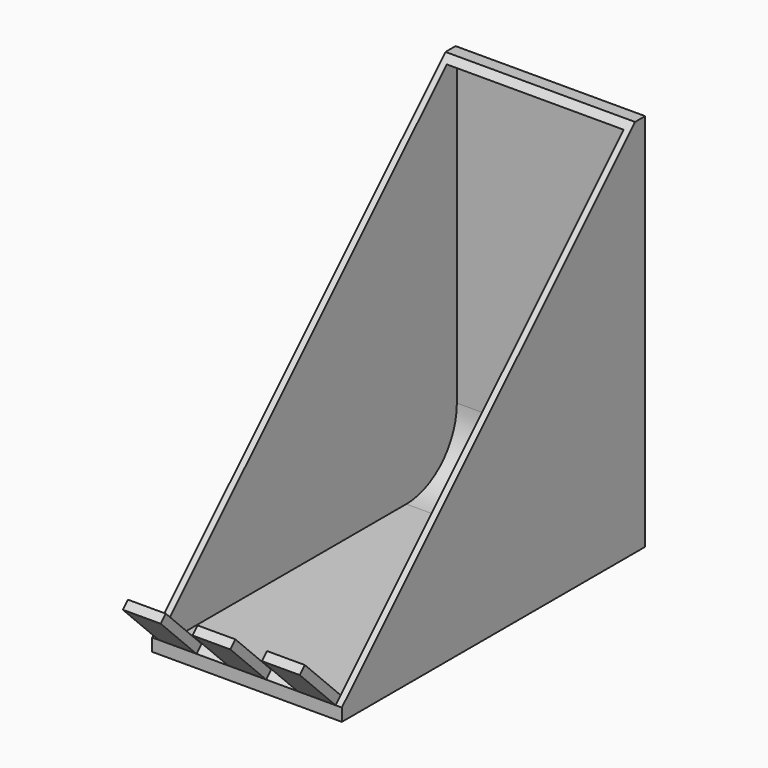
from build123d import *

# Parameters (mm, degrees)
F0_W     = 76.2
F0_H     = 152.4
F1_DEPTH = 152.4
F2_SIZE  = 147.32
F3_T     = -2.54
F4_R     = 25.4
F5_R     = 5.07999
F6_W     = 15.24
F6_H     = 3.5921024484
F7_DEPTH = 25.4


# Not quite as in the source:
# - a fillet or chamfer is up to 0.001 mm smaller than in the source, because OpenCascade refuses the exact size


with BuildPart() as f1:
    # F0 (on Top) → F1 (new body)
    with BuildSketch(Plane.XY):
        Rectangle(F0_W, F0_H)
    extrude(amount=F1_DEPTH)

    # F2
    f2_edges = [f1.edges().sort_by_distance(p)[0] for p in [
        (0, -76.2, 152.4),
    ]]
    chamfer(f2_edges, length=F2_SIZE)

    # F3
    f3_openings = [f1.faces().sort_by_distance(p)[0] for p in [
        (0, -2.54, 78.74),
    ]]
    offset(amount=F3_T, openings=f3_openings)

    # F4
    f4_edges = [f1.edges().sort_by_distance(p)[0] for p in [
        (0, 73.66, 2.54),
    ]]
    fillet(f4_edges, radius=F4_R)

    # F5 (radius 5.08 in the source; OpenCascade refuses exactly that, so slightly less here)
    f5_edges = [f1.edges().sort_by_distance(p)[0] for p in [
        (0, -73.66, 2.54),
    ]]
    fillet(f5_edges, radius=F5_R)

    # F6 (on face) → F7 (join)
    with BuildSketch(Plane(origin=(0, -40.64, 40.64), x_dir=(1, 0, 0), z_dir=(0, -0.7071067812, 0.7071067812))):
        with Locations((-27.94, -48.4933830538)):
            Rectangle(F6_W, F6_H)
        with Locations((27.94, -48.4933830538)):
            Rectangle(F6_W, F6_H)
        with Locations((0.0408754674, -48.4933830538)):
            Rectangle(F6_W, F6_H)
    extrude(amount=F7_DEPTH)


solid = f1.part
